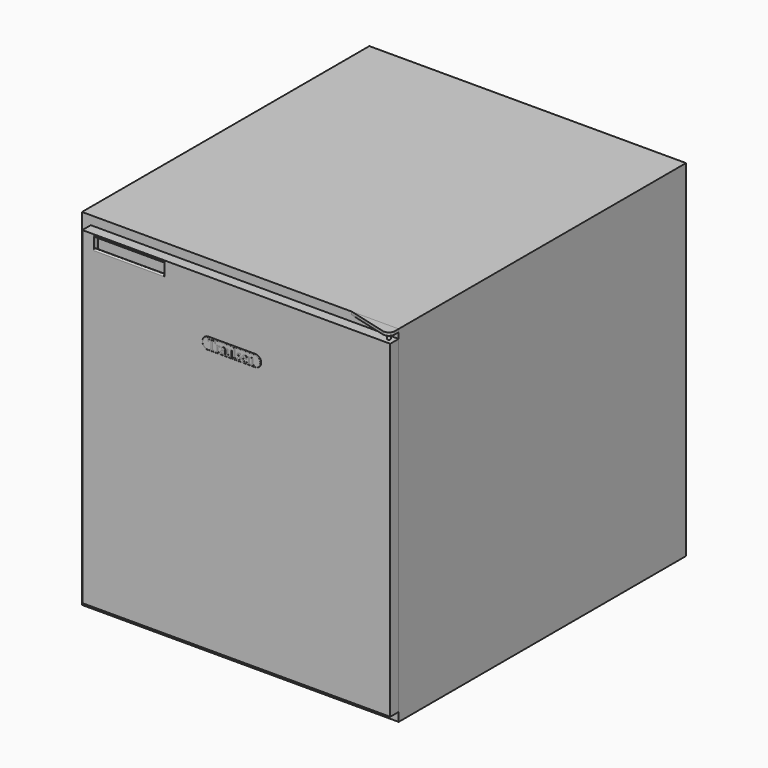
from build123d import *

# Parameters (mm, degrees)
F0_W          = 685.8
F0_H          = 749.3
F0_W_2        = 609.6
F0_H_2        = 673.1
F1_DEPTH      = 777.875
F2_W          = 685.8
F2_H          = 749.3
F3_DEPTH      = 25.4
F4_W          = 595.7696102142
F4_H          = 3.175
F5_DEPTH      = 762
F4_W_2        = 609.6
F6_W          = 666.75
F6_H          = 711.2
F7_DEPTH      = 22.86
F9_DEPTH      = 6.35
F10_R         = 3.175
F11_DEPTH     = 25.4
F12_R         = 3.175
F13_DEPTH     = 12.7
F16_DEPTH     = 152.4
F18_DEPTH     = 152.4
F19_R         = 3.17499
F21_DEPTH     = 1.5875
F22_R         = 1.58749
F23_TEXT_SIZE = 28.6631944444
F24_DEPTH     = 0.254


# Not quite as in the source:
# - a fillet or chamfer is up to 0.001 mm smaller than in the source, because OpenCascade refuses the exact size
# - Text() gives the source's letters only with a copy of the font that has no kerning and outlines rounded to 1/6400 em; it was checked with that copy


with BuildPart() as f1:
    # F0 (on Front) → F1 (new body)
    with BuildSketch(Plane.XZ):
        Rectangle(F0_W, F0_H)
        Rectangle(F0_W_2, F0_H_2, mode=Mode.SUBTRACT)
    extrude(amount=-F1_DEPTH)

    # F2 (on face) → F3 (join)
    with BuildSketch(Plane(origin=(0, 777.875, 0), x_dir=(-1, 0, 0), z_dir=(0, 1, 0))):
        Rectangle(F2_W, F2_H)
    extrude(amount=-F3_DEPTH)


with BuildPart() as f5:
    # F4 (on face) → F5 (new body)
    with BuildSketch(Plane.XZ.offset(-752.475)):
        with Locations((-6.9151948929, 106.3625)):
            Rectangle(F4_W, F4_H)
    extrude(amount=F5_DEPTH)


with BuildPart() as f5b:
    # F4 (on face) → F5, piece 2 (new body)
    with BuildSketch(Plane.XZ.offset(-752.475)):
        with Locations((0, -125.4125)):
            Rectangle(F4_W_2, F4_H)
    extrude(amount=F5_DEPTH)


with BuildPart() as f7:
    # F6 (on face) → F7 (new body)
    with BuildSketch(Plane.XZ):
        with Locations((9.525, 0)):
            Rectangle(F6_W, F6_H)
    extrude(amount=F7_DEPTH)

    # F12 (on face) → F13 (cut)
    with BuildSketch(Plane.XY.offset(355.6)):
        with Locations((330.2, -10.5897769011)):
            Circle(F12_R)
    extrude(amount=-F13_DEPTH, mode=Mode.SUBTRACT)

    # F15 (on offset) → F16 (cut)
    with BuildSketch(Plane(origin=(-298.45, 0, 0), x_dir=(0, -1, 0), z_dir=(-1, 0, 0))):
        Polygon((22.86, 327.025), (22.86, 352.425), (10.16, 352.425), (10.16, 314.325), (19.685, 314.325), (19.685, 327.025), align=None)
    extrude(amount=-F16_DEPTH, mode=Mode.SUBTRACT)


with BuildPart() as f9:
    # F8 (on face) → F9 (new body)
    with BuildSketch(Plane.XY.offset(374.65)):
        with BuildLine():
            Line((342.9, 0), (241.3, 0))
            Line((241.3, 0), (326.9240840816, -22.86))
            ThreePointArc((326.9240840816, -22.86), (337.9358214766, -20.6618703321), (342.9, -10.5897769011))
            Line((342.9, -10.5897769011), (342.9, 0))
        make_face()
    extrude(amount=-F9_DEPTH)

    # F10 (on face) → F11 (join)
    with BuildSketch(Plane(origin=(0, 0, 368.3), x_dir=(1, 0, 0), z_dir=(0, 0, -1))):
        with Locations((330.2, 10.5897769011)):
            Circle(F10_R)
    extrude(amount=F11_DEPTH)


with BuildPart() as f18:
    # F17 (on offset) → F18 (new body)
    with BuildSketch(Plane(origin=(-298.45, 0, 0), x_dir=(0, -1, 0), z_dir=(-1, 0, 0))):
        Polygon((22.86, 354.0125), (22.86, 352.425), (10.16, 352.425), (10.16, 314.325), (19.685, 314.325), (19.685, 327.025), (22.86, 327.025), (22.86, 325.4375), (24.4475, 325.4375), (24.4475, 328.6125), (18.0975, 328.6125), (18.0975, 315.9125), (11.7475, 315.9125), (11.7475, 350.8375), (22.86, 350.8375), (24.4475, 350.8375), (24.4475, 354.0125), align=None)
    extrude(amount=-F18_DEPTH)

    # F19 (radius 3.175 in the source; OpenCascade refuses exactly that, so slightly less here)
    f19_edges = [f18.edges().sort_by_distance(p)[0] for p in [
        (-222.25, -24.4475, 350.8375),
        (-222.25, -24.4475, 328.6125),
        (-222.25, -18.0975, 328.6125),
        (-222.25, -11.7475, 350.8375),
    ]]
    fillet(f19_edges, radius=F19_R)


with BuildPart() as f21:
    # F20 (on face) → F21 (new body)
    with BuildSketch(Plane.XZ.offset(22.86)):
        with BuildLine():
            ThreePointArc((-50.8, 241.3), (-63.5, 228.6), (-50.8, 215.9))
            Line((-50.8, 215.9), (50.8, 215.9))
            ThreePointArc((50.8, 215.9), (63.5, 228.6), (50.8, 241.3))
            Line((50.8, 241.3), (-50.8, 241.3))
        make_face()
    extrude(amount=F21_DEPTH)

    # F22 (radius 1.5875 in the source; OpenCascade refuses exactly that, so slightly less here)
    f22_edges = [f21.edges().sort_by_distance(p)[0] for p in [
        (-63.5, -24.4475, 228.6),
        (0, -24.4475, 215.9),
        (63.5, -24.4475, 228.6),
        (0, -24.4475, 241.3),
    ]]
    fillet(f22_edges, radius=F22_R)


with BuildPart() as f24:
    # F23 (on face) → F24 (new body)
    with BuildSketch(Plane.XZ.offset(24.4475)):
        with Locations((-50.8189480252, 219.075)):
            Text('Traulsen', F23_TEXT_SIZE, font='Tinos', text_align=(TextAlign.LEFT, TextAlign.BOTTOM))
    extrude(amount=F24_DEPTH)


solid = Compound([f1.part, f5.part, f5b.part, f7.part, f9.part, f18.part, f21.part, f24.part])
